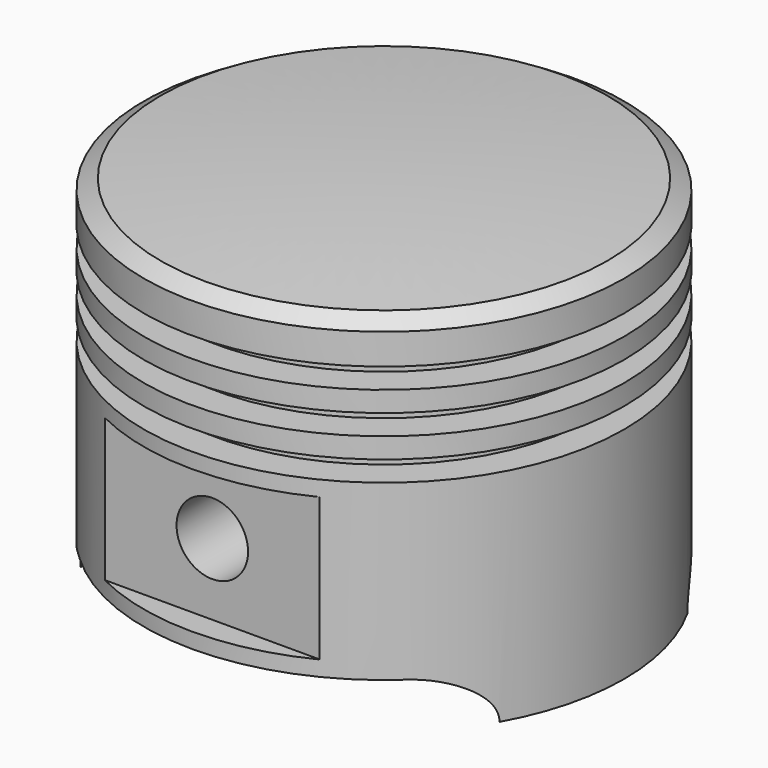
from build123d import *

# Parameters (mm, degrees)
F2_R     = 7
F3_DEPTH = 72
F5_START = 42
F4_W     = 42
F4_H     = 28
F4_R     = 7
F5_DEPTH = 28.7
F9_DEPTH = 211.3


# Not quite as in the source:
# - a pattern or mirror of a feature is missing from the dataset's text; its kind, count and spacing are read off the source's solid


with BuildPart() as f1:
    # F0 (on Front) → F1 (revolve)
    with BuildSketch(Plane.XZ):
        with BuildLine():
            Line((47, 87), (43.7432713807, 89))
            ThreePointArc((43.7432713807, 89), (21.8944844144, 90.4997389679), (0, 91))
            Line((0, 91), (0, 18))
            Line((0, 18), (47, 18))
            Line((47, 18), (47, 33))
            Line((47, 33), (47, 57))
            Line((47, 57), (47, 61))
            Line((47, 61), (41, 61))
            Line((41, 61), (41, 65))
            Line((41, 65), (47, 65))
            Line((47, 65), (47, 69))
            Line((47, 69), (41, 69))
            Line((41, 69), (41, 73))
            Line((41, 73), (47, 73))
            Line((47, 73), (47, 77))
            Line((47, 77), (41, 77))
            Line((41, 77), (41, 81))
            Line((41, 81), (47, 81))
            Line((47, 81), (47, 87))
        make_face()
    revolve(axis=Axis((0, 0, 45.5), (0, 0, -1)))

    # F2 (on Front) → F3 (cut, symmetric)
    with BuildSketch(Plane.XZ):
        with Locations((0, 44)):
            Circle(F2_R)
    extrude(amount=F3_DEPTH, both=True, mode=Mode.SUBTRACT)

    # F4 (on Front) → F5 (cut)
    with BuildSketch(Plane.XZ.offset(F5_START)):
        with Locations((0, 44)):
            Rectangle(F4_W, F4_H)
        with Locations((0, 44)):
            Circle(F4_R, mode=Mode.SUBTRACT)
    f5 = extrude(amount=F5_DEPTH, mode=Mode.SUBTRACT)

    # F5_copies: F5 across plane
    add(f5.mirror(Plane.ZX), mode=Mode.SUBTRACT)

    # F6 (on Front) → F7 (revolve, cut)
    with BuildSketch(Plane.XZ):
        with BuildLine():
            Line((0, 81), (0, 18))
            Line((0, 18), (43, 18))
            Line((43, 18), (43, 26))
            Line((43, 26), (25, 33))
            Line((25, 33), (25, 57))
            Line((25, 57), (28, 57))
            ThreePointArc((28, 57), (33.6568542495, 59.3431457505), (36, 65))
            Line((36, 65), (36, 81))
            Line((36, 81), (0, 81))
        make_face()
    revolve(axis=Axis((0, 0, 34.176344052), (0, 0, 1)), mode=Mode.SUBTRACT)

    # F8 (on Front) → F9 (cut, symmetric)
    with BuildSketch(Plane.XZ):
        with BuildLine():
            Line((32, 27), (-32, 27))
            ThreePointArc((-32, 27), (-38.3639610307, 24.3639610307), (-41, 18))
            Line((-41, 18), (41, 18))
            ThreePointArc((41, 18), (38.3639610307, 24.3639610307), (32, 27))
        make_face()
    extrude(amount=F9_DEPTH, both=True, mode=Mode.SUBTRACT)


solid = f1.part
